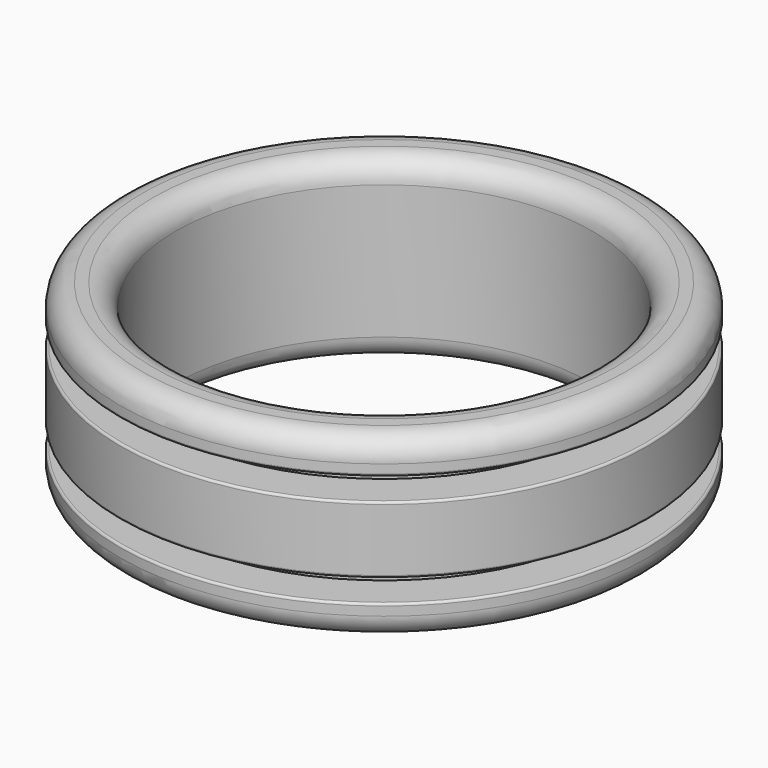
from build123d import *

# Parameters (mm, degrees)
F2_R = 2.54
F3_R = 0.254


# Not quite as in the source:
# - a feature of the source that left no trace in its solid (it failed there, or was rolled back) is left out


with BuildPart() as f1:
    # F0 (on Front) → F1 (revolve)
    with BuildSketch(Plane.XZ):
        Polygon((61.408632046, 23.7112408589), (61.408632046, 27.5212408589), (55.058632046, 27.5212408589), (55.058632046, 7.2012408589), (61.408632046, 7.2012408589), (61.408632046, 11.0112408589), (56.963632046, 11.0112408589), (56.963632046, 13.5512408589), (61.408632046, 13.5512408589), (61.408632046, 21.1712408589), (56.963632046, 21.1712408589), (56.963632046, 23.7112408589), align=None)
    revolve(axis=Axis((31.3779890053, 0, 18.6312408589), (0, 0, -1)))

    # F2
    f2_edges = [f1.edges().sort_by_distance(p)[0] for p in [
        (1.347346, 0, 27.521241),
        (7.697346, 0, 27.521241),
        (7.697346, 0, 7.201241),
        (1.347346, 0, 7.201241),
    ]]
    fillet(f2_edges, radius=F2_R)

    # F3
    f3_edges = [f1.edges().sort_by_distance(p)[0] for p in [
        (1.347346, 0, 21.171241),
        (1.347346, 0, 23.711241),
        (1.347346, 0, 13.551241),
        (1.347346, 0, 11.011241),
    ]]
    fillet(f3_edges, radius=F3_R)


solid = f1.part
